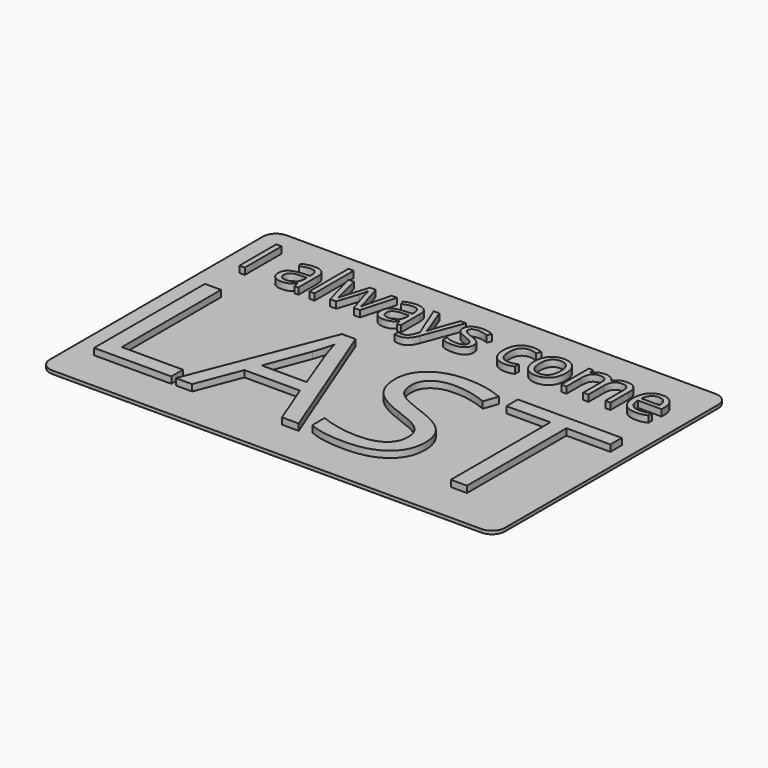
from build123d import *

# Parameters (mm, degrees)
F0_W           = 70
F0_H           = 45
F1_DEPTH       = 0.5
F2_R           = 2
F3_TEXT_SIZE   = 29.8611111111
F3_TEXT_SIZE_2 = 9.9160951371
F4_DEPTH       = 1


# Not quite as in the source:
# - Text() gives the source's letters only with a copy of the font that has no kerning and outlines rounded to 1/6400 em; it was checked with that copy


with BuildPart() as f1:
    # F0 (on Top) → F1 (new body)
    with BuildSketch(Plane.XY):
        with Locations((14.7194565833, -16.0120362043)):
            Rectangle(F0_W, F0_H)
    extrude(amount=-F1_DEPTH)

    # F2
    f2_edges = [f1.edges().sort_by_distance(p)[0] for p in [
        (49.719457, -38.512036, -0.25),
        (-20.280543, -38.512036, -0.25),
        (-20.280543, 6.487964, -0.25),
        (49.719457, 6.487964, -0.25),
    ]]
    fillet(f2_edges, radius=F2_R)


with BuildPart() as f4:
    # F3 (on Top) → F4 (new body)
    with BuildSketch(Plane.XY):
        with Locations((-19.7631280522, -32.3042826562)):
            Text('LAST', F3_TEXT_SIZE, font='Open Sans', text_align=(TextAlign.LEFT, TextAlign.BOTTOM))
        with Locations((-17.5388404098, -4.6897000866)):
            Text('I always come', F3_TEXT_SIZE_2, font='Open Sans', text_align=(TextAlign.LEFT, TextAlign.BOTTOM))
    extrude(amount=F4_DEPTH)


solid = Compound([f1.part, f4.part])
